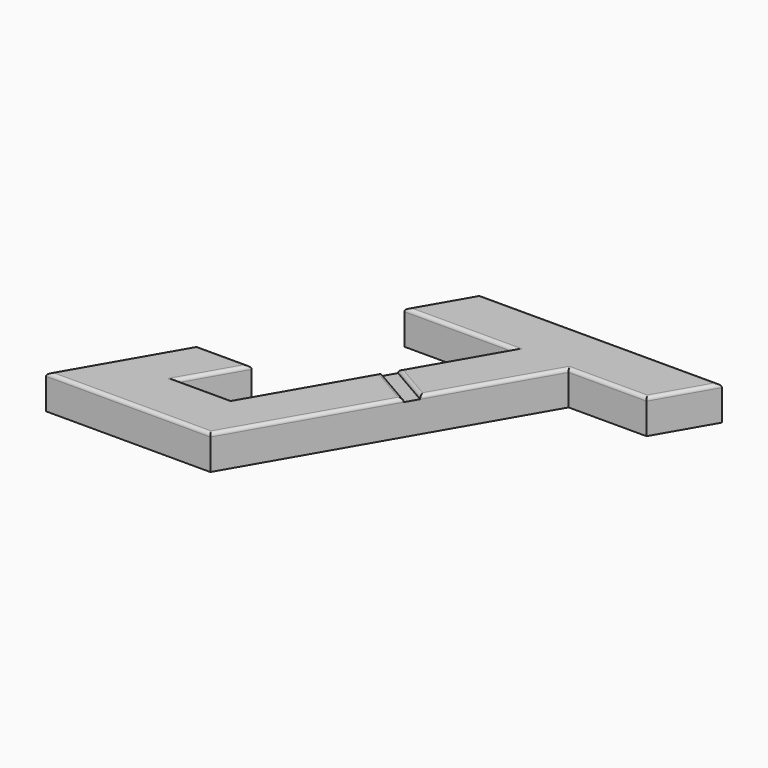
from build123d import *

# Parameters (mm, degrees)
F1_DEPTH = 2.5
F4_W     = 1
F4_H     = 5.3799478337
F5_DEPTH = 100
F6_T     = -0.75
F7_R     = 0.24999
F9_DEPTH = 1.75


# Not quite as in the source:
# - a fillet or chamfer is up to 0.001 mm smaller than in the source, because OpenCascade refuses the exact size


with BuildPart() as f1:
    # F0 (on Top) → F1 (new body)
    with BuildSketch(Plane.XY):
        Polygon((-7.6905989232, 19), (-10, 15), (-2, 15), (-10.6602540378, 0), (-14.6602540378, 0), (-12.3508529611, 4), (-16.3508529611, 4), (-20.9696551146, -4), (-8.9696551146, -4), (2, 15), (7.6905989232, 15), (10, 19), align=None)
    extrude(amount=F1_DEPTH)

    # F4 (on offset) → F5 (cut)
    with BuildSketch(Plane(origin=(16.6554445662, -9.6160254038, 0), x_dir=(0.5, 0.8660254038, 0), z_dir=(0.8660254038, -0.5, 0))):
        with Locations((4.397114317, 4.9399739169)):
            Rectangle(F4_W, F4_H)
    extrude(amount=-F5_DEPTH, mode=Mode.SUBTRACT)

    # F6
    f6_openings = [f1.faces().sort_by_distance(p)[0] for p in [
        (-8.51122, 16.807119, 0),
    ]]
    offset(amount=F6_T, openings=f6_openings, kind=Kind.INTERSECTION)

    # F7 (radius 0.25 in the source; OpenCascade refuses exactly that, so slightly less here)
    f7_edges = [f1.edges().sort_by_distance(p)[0] for p in [
        (-0.273317, 11.0625, 2.5),
        (4.845299, 15, 2.5),
        (8.845299, 17, 2.5),
        (1.154701, 19, 2.5),
        (-8.845299, 17, 2.5),
        (-6, 15, 2.5),
        (-3.773317, 11.928525, 2.5),
        (-4.046633, 7.991025, 2.5),
        (-8.353444, 3.995513, 2.5),
        (-12.660254, 0, 2.5),
        (-13.505553, 2, 2.5),
        (-14.350853, 4, 2.5),
        (-18.660254, 0, 2.5),
        (-14.969655, -4, 2.5),
        (-6.008144, 1.129487, 2.5),
        (-4.546633, 7.125, 2.5),
    ]]
    fillet(f7_edges, radius=F7_R)

    # F8 (on face) → F9 (join, through all)
    with BuildSketch(Plane(origin=(0, 0, 1.75), x_dir=(1, 0, 0), z_dir=(0, 0, -1))):
        Polygon((-4.3476606357, -15.75), (-5.2575862213, -18.25), (-3.2575862213, -18.25), (-2.3476606357, -15.75), align=None)
        Polygon((3.2575862213, -15.75), (2.3476606357, -18.25), (4.3476606357, -18.25), (5.2575862213, -15.75), align=None)
    extrude(amount=F9_DEPTH)


solid = f1.part
